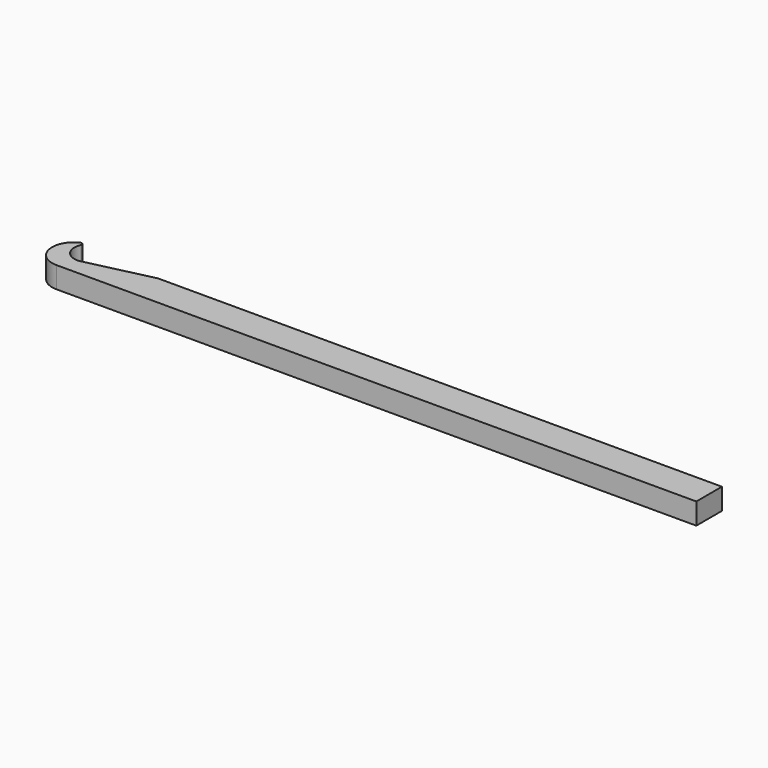
from build123d import *

# Parameters (mm, degrees)
F1_DEPTH = 2
F2_R     = 0.2


with BuildPart() as f1:
    # F0 (on Top) → F1 (new body)
    with BuildSketch(Plane.XY):
        with BuildLine():
            ThreePointArc((2.0172090196, 1.8148367186), (1.3567207288, 0.5204837279), (0, 0))
            Line((0, 0), (60, 0))
            Line((60, 0), (60, 3))
            Line((60, 3), (7.1340496652, 3))
            Line((7.1340496652, 3), (2.0172090196, 1.8148367186))
        make_face()
        with BuildLine():
            ThreePointArc((-0.286715437, 4.0366195626), (-2.023394625, 1.8847733915), (0, 0))
            Line((0, 0), (0, 1.744815443))
            ThreePointArc((0, 1.744815443), (-0.710712171, 2.8197388016), (-0.286715437, 4.0366195626))
        make_face()
        with BuildLine():
            Line((0, 1.744815443), (0, 0))
            ThreePointArc((0, 0), (1.3567207288, 0.5204837279), (2.0172090196, 1.8148367186))
            Line((2.0172090196, 1.8148367186), (1.1959759108, 1.6246226015))
            ThreePointArc((1.1959759108, 1.6246226015), (1.0578352718, 1.5853362888), (0.9164894863, 1.5598879203))
            ThreePointArc((0.9164894863, 1.5598879203), (0.4429542769, 1.5765730666), (0, 1.744815443))
        make_face()
    extrude(amount=F1_DEPTH)

    # F2
    f2_edges = [f1.edges().sort_by_distance(p)[0] for p in [
        (-0.286715, 4.03662, 1),
    ]]
    fillet(f2_edges, radius=F2_R)


solid = f1.part
